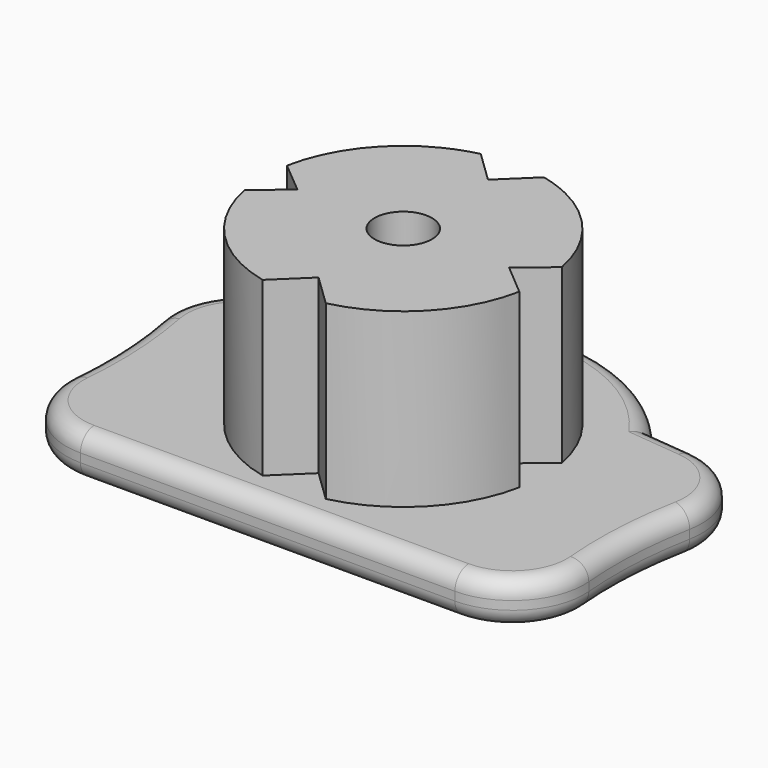
from build123d import *

# Parameters (mm, degrees)
F0_R     = 2
F1_DEPTH = 15
F2_DEPTH = 3
F3_R     = 5
F4_R     = 5
F5_R     = 1.2


with BuildPart() as f1:
    # F0 (on Top) → F1 (new body)
    with BuildSketch(Plane.XY):
        with BuildLine():
            Line((9.5707826587, -1.8608114628), (7.3763099499, 0))
            ThreePointArc((7.3763099499, 0), (5.2158387857, -5.2158387857), (0, -7.3763099499))
            Line((0, -7.3763099499), (2.2002961183, -9.4984839312))
            ThreePointArc((2.2002961183, -9.4984839312), (7.0159164816, -6.770481218), (9.5707826587, -1.8608114628))
        make_face()
        with BuildLine():
            ThreePointArc((0, -7.3763099499), (5.2158387857, -5.2158387857), (7.3763099499, 0))
            ThreePointArc((7.3763099499, 0), (5.2158387857, 5.2158387857), (0, 7.3763099499))
            ThreePointArc((0, 7.3763099499), (-5.2158387857, 5.2158387857), (-7.3763099499, 0))
            ThreePointArc((-7.3763099499, 0), (-5.2158387857, -5.2158387857), (0, -7.3763099499))
        make_face()
        Circle(F0_R, mode=Mode.SUBTRACT)
        with BuildLine():
            ThreePointArc((9.5742217065, 1.8430351908), (7.7357792995, 5.9346624697), (4.2599529151, 8.7701368952))
            Line((4.2599529151, 8.7701368952), (1.7095643673, 9.02517575))
            Line((1.7095643673, 9.02517575), (0, 7.3763099499))
            ThreePointArc((0, 7.3763099499), (5.2158387857, 5.2158387857), (7.3763099499, 0))
            Line((7.3763099499, 0), (9.5742217065, 1.8430351908))
        make_face()
        with BuildLine():
            Line((1.7095643673, 9.02517575), (4.2599529151, 8.7701368952))
            ThreePointArc((4.2599529151, 8.7701368952), (3.2505886766, 9.1921800056), (2.2002961183, 9.4984839312))
            Line((2.2002961183, 9.4984839312), (1.7095643673, 9.02517575))
        make_face()
        with BuildLine():
            Line((-1.7095643673, 9.02517575), (-4.2599529151, 8.7701368952))
            ThreePointArc((-4.2599529151, 8.7701368952), (-7.7357792995, 5.9346624697), (-9.5742217065, 1.8430351908))
            Line((-9.5742217065, 1.8430351908), (-7.3763099499, 0))
            ThreePointArc((-7.3763099499, 0), (-5.2158387857, 5.2158387857), (0, 7.3763099499))
            Line((0, 7.3763099499), (-1.7095643673, 9.02517575))
        make_face()
        with BuildLine():
            ThreePointArc((-2.2002961183, 9.4984839312), (-3.2505886766, 9.1921800056), (-4.2599529151, 8.7701368952))
            Line((-4.2599529151, 8.7701368952), (-1.7095643673, 9.02517575))
            Line((-1.7095643673, 9.02517575), (-2.2002961183, 9.4984839312))
        make_face()
        with BuildLine():
            Line((-7.3763099499, 0), (-9.5707826587, -1.8608114628))
            ThreePointArc((-9.5707826587, -1.8608114628), (-7.0159164816, -6.770481218), (-2.2002961183, -9.4984839312))
            Line((-2.2002961183, -9.4984839312), (0, -7.3763099499))
            ThreePointArc((0, -7.3763099499), (-5.2158387857, -5.2158387857), (-7.3763099499, 0))
        make_face()
    extrude(amount=F1_DEPTH)

    # F0 (on Top) → F2 (join)
    with BuildSketch(Plane.XY):
        with BuildLine():
            Line((4.2599529151, 8.7701368952), (10.7868960269, 8.1174425841))
            ThreePointArc((10.7868960269, 8.1174425841), (0, 13.5), (-10.7868960269, 8.1174425841))
            Line((-10.7868960269, 8.1174425841), (-4.2599529151, 8.7701368952))
            ThreePointArc((-4.2599529151, 8.7701368952), (-3.2505886766, 9.1921800056), (-2.2002961183, 9.4984839312))
            ThreePointArc((-2.2002961183, 9.4984839312), (0, 9.75), (2.2002961183, 9.4984839312))
            ThreePointArc((2.2002961183, 9.4984839312), (3.2505886766, 9.1921800056), (4.2599529151, 8.7701368952))
        make_face()
        Polygon((0, 7.3763099499), (1.7095643673, 9.02517575), (0, 9.1961321867), (-1.7095643673, 9.02517575), align=None)
        with BuildLine():
            Line((1.7095643673, 9.02517575), (2.2002961183, 9.4984839312))
            ThreePointArc((2.2002961183, 9.4984839312), (0, 9.75), (-2.2002961183, 9.4984839312))
            Line((-2.2002961183, 9.4984839312), (-1.7095643673, 9.02517575))
            Line((-1.7095643673, 9.02517575), (0, 9.1961321867))
            Line((0, 9.1961321867), (1.7095643673, 9.02517575))
        make_face()
        with BuildLine():
            ThreePointArc((8.2654431298, -10.6739144585), (12.1209216286, -5.9441785701), (13.5, 0))
            ThreePointArc((13.5, 0), (12.8037708579, 4.2794219024), (10.7868960269, 8.1174425841))
            Line((10.7868960269, 8.1174425841), (4.2599529151, 8.7701368952))
            ThreePointArc((4.2599529151, 8.7701368952), (7.7357792995, 5.9346624697), (9.5742217065, 1.8430351908))
            ThreePointArc((9.5742217065, 1.8430351908), (9.7059559457, 0.9256992928), (9.75, 0))
            ThreePointArc((9.75, 0), (9.7050922438, -0.9347109387), (9.5707826587, -1.8608114628))
            ThreePointArc((9.5707826587, -1.8608114628), (7.0159164816, -6.770481218), (2.2002961183, -9.4984839312))
            ThreePointArc((2.2002961183, -9.4984839312), (0, -9.75), (-2.2002961183, -9.4984839312))
            ThreePointArc((-2.2002961183, -9.4984839312), (-7.0159164816, -6.770481218), (-9.5707826587, -1.8608114628))
            ThreePointArc((-9.5707826587, -1.8608114628), (-9.7499957971, -0.0090529401), (-9.5742217065, 1.8430351908))
            ThreePointArc((-9.5742217065, 1.8430351908), (-7.7357792995, 5.9346624697), (-4.2599529151, 8.7701368952))
            Line((-4.2599529151, 8.7701368952), (-10.7868960269, 8.1174425841))
            ThreePointArc((-10.7868960269, 8.1174425841), (-13.3800852655, -1.7953602115), (-8.2654431298, -10.6739144585))
            Line((-8.2654431298, -10.6739144585), (0, -9.8038678133))
            Line((0, -9.8038678133), (8.2654431298, -10.6739144585))
        make_face()
        with BuildLine():
            ThreePointArc((-8.2654431298, -10.6739144585), (-13.3800852655, -1.7953602115), (-10.7868960269, 8.1174425841))
            Line((-10.7868960269, 8.1174425841), (-20, 7.1961321867))
            ThreePointArc((-20, 7.1961321867), (-17.9538534771, -2.2224916805), (-19, -11.8038678133))
            Line((-19, -11.8038678133), (-8.2654431298, -10.6739144585))
        make_face()
        with BuildLine():
            ThreePointArc((-6.5512368792, -11.8038678133), (-7.4298519681, -11.2715260605), (-8.2654431298, -10.6739144585))
            Line((-8.2654431298, -10.6739144585), (-19, -11.8038678133))
            Line((-19, -11.8038678133), (-6.5512368792, -11.8038678133))
        make_face()
        with BuildLine():
            Line((19, -11.8038678133), (8.2654431298, -10.6739144585))
            ThreePointArc((8.2654431298, -10.6739144585), (7.4298519681, -11.2715260605), (6.5512368792, -11.8038678133))
            Line((6.5512368792, -11.8038678133), (19, -11.8038678133))
        make_face()
        with BuildLine():
            ThreePointArc((6.5512368792, -11.8038678133), (7.4298519681, -11.2715260605), (8.2654431298, -10.6739144585))
            Line((8.2654431298, -10.6739144585), (0, -9.8038678133))
            Line((0, -9.8038678133), (-8.2654431298, -10.6739144585))
            ThreePointArc((-8.2654431298, -10.6739144585), (-7.4298519681, -11.2715260605), (-6.5512368792, -11.8038678133))
            Line((-6.5512368792, -11.8038678133), (6.5512368792, -11.8038678133))
        make_face()
        with BuildLine():
            ThreePointArc((10.7868960269, 8.1174425841), (12.8037708579, 4.2794219024), (13.5, 0))
            ThreePointArc((13.5, 0), (12.1209216286, -5.9441785701), (8.2654431298, -10.6739144585))
            Line((8.2654431298, -10.6739144585), (19, -11.8038678133))
            ThreePointArc((19, -11.8038678133), (17.9538534771, -2.2224916805), (20, 7.1961321867))
            Line((20, 7.1961321867), (10.7868960269, 8.1174425841))
        make_face()
        with BuildLine():
            ThreePointArc((9.75, 0), (9.7059559457, 0.9256992928), (9.5742217065, 1.8430351908))
            Line((9.5742217065, 1.8430351908), (7.3763099499, 0))
            Line((7.3763099499, 0), (9.5707826587, -1.8608114628))
            ThreePointArc((9.5707826587, -1.8608114628), (9.7050922438, -0.9347109387), (9.75, 0))
        make_face()
        with BuildLine():
            Line((-7.3763099499, 0), (-9.5742217065, 1.8430351908))
            ThreePointArc((-9.5742217065, 1.8430351908), (-9.7499957971, -0.0090529401), (-9.5707826587, -1.8608114628))
            Line((-9.5707826587, -1.8608114628), (-7.3763099499, 0))
        make_face()
        with BuildLine():
            Line((2.2002961183, -9.4984839312), (0, -7.3763099499))
            Line((0, -7.3763099499), (-2.2002961183, -9.4984839312))
            ThreePointArc((-2.2002961183, -9.4984839312), (0, -9.75), (2.2002961183, -9.4984839312))
        make_face()
    extrude(amount=F2_DEPTH)

    # F3
    f3_edges = [f1.edges().sort_by_distance(p)[0] for p in [
        (19, -11.803868, 1.5),
    ]]
    fillet(f3_edges, radius=F3_R)

    # F4
    f4_edges = [f1.edges().sort_by_distance(p)[0] for p in [
        (-19, -11.803868, 1.5),
        (20, 7.196132, 1.5),
        (-20, 7.196132, 1.5),
    ]]
    fillet(f4_edges, radius=F4_R)

    # F5
    f5_edges = [f1.edges().sort_by_distance(p)[0] for p in [
        (0, -11.803868, 3),
        (0, 13.5, 3),
        (0, -11.803868, 0),
        (0, 13.5, 0),
    ]]
    fillet(f5_edges, radius=F5_R)


solid = f1.part
